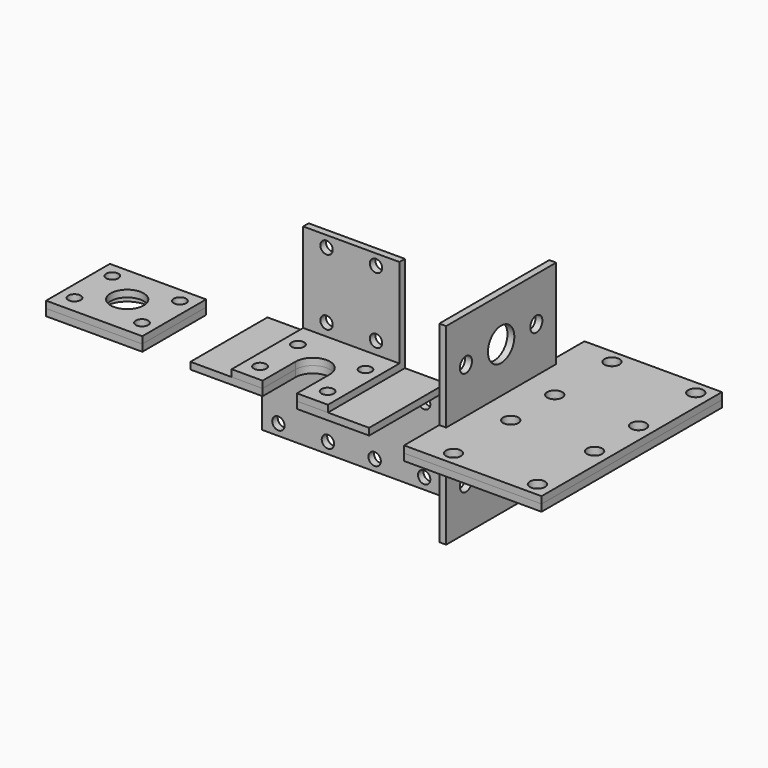
from build123d import *

# Parameters (mm, degrees)
F1_W      = 32.5
F1_H      = 2.5
F1_W_2    = 2.5
F2_DEPTH  = 17.5
F1_H_2    = 32.5
F3_DEPTH  = 17.5
F4_W      = 32.5
F4_H      = 2.5
F4_W_2    = 2.5
F5_DEPTH  = 32.5
F4_H_2    = 32.5
F6_DEPTH  = 32.5
F7_R      = 2.25
F8_DEPTH  = 5
F9_DEPTH  = 5
F11_R     = 2.25
F12_DEPTH = 5
F10_W     = 35
F10_H     = 29
F10_R     = 2.25
F13_DEPTH = 2.5
F14_DEPTH = 2.5
F15_W     = 2.5
F15_H     = 32.5
F15_H_2   = 2.5
F16_DEPTH = 25
F15_W_2   = 47.5
F17_DEPTH = 41
F18_DEPTH = 41
F19_DEPTH = 25
F20_R     = 2.75
F20_R_2   = 6
F21_DEPTH = 2.5
F22_DEPTH = 5
F23_R     = 2.75
F24_DEPTH = 5


with BuildPart() as f2:
    # F1 (on Right) → F2 (new body, symmetric)
    with BuildSketch(Plane.YZ):
        with Locations((-18.75, 1.25)):
            Rectangle(F1_W, F1_H)
        with Locations((-1.25, 1.25)):
            Rectangle(F1_W_2, F1_H)
    extrude(amount=F2_DEPTH, both=True)

    # F1 (on Right) → F3 (join, symmetric)
    with BuildSketch(Plane.YZ):
        with Locations((-1.25, 1.25)):
            Rectangle(F1_W_2, F1_H)
        with Locations((-1.25, 18.75)):
            Rectangle(F1_W_2, F1_H_2)
    extrude(amount=F3_DEPTH, both=True)

    # F7 (on Front) → F8 (cut, symmetric)
    with BuildSketch(Plane.XZ):
        with Locations((9, 31)):
            Circle(F7_R)
        with Locations((9, 7)):
            Circle(F7_R)
        with Locations((-9, 7)):
            Circle(F7_R)
        with Locations((-9, 31)):
            Circle(F7_R)
    extrude(amount=F8_DEPTH, both=True, mode=Mode.SUBTRACT)


with BuildPart() as f5:
    # F4 (on Right) → F5 (new body, symmetric)
    with BuildSketch(Plane.YZ):
        with Locations((-18.75, -1.25)):
            Rectangle(F4_W, F4_H)
        with Locations((-1.25, -1.25)):
            Rectangle(F4_W_2, F4_H)
    extrude(amount=F5_DEPTH, both=True)

    # F4 (on Right) → F6 (join, symmetric)
    with BuildSketch(Plane.YZ):
        with Locations((-1.25, -18.75)):
            Rectangle(F4_W_2, F4_H_2)
        with Locations((-1.25, -1.25)):
            Rectangle(F4_W_2, F4_H)
    extrude(amount=F6_DEPTH, both=True)

    # F7 (on Front) → F9 (cut, symmetric)
    with BuildSketch(Plane.XZ):
        with Locations((26.5, -7)):
            Circle(F7_R)
        with Locations((8.5, -7)):
            Circle(F7_R)
        with Locations((-8.5, -7)):
            Circle(F7_R)
        with Locations((-26.5, -7)):
            Circle(F7_R)
        with Locations((-26.5, -31)):
            Circle(F7_R)
        with Locations((-8.5, -31)):
            Circle(F7_R)
        with Locations((8.5, -31)):
            Circle(F7_R)
        with Locations((26.5, -31)):
            Circle(F7_R)
    extrude(amount=F9_DEPTH, both=True, mode=Mode.SUBTRACT)


with BuildPart() as f12_tool:
    # F11 (on Top) → F12 (new body, symmetric)
    with BuildSketch(Plane.XY):
        with BuildLine():
            ThreePointArc((-6.25, -20), (0, -26.25), (6.25, -20))
            ThreePointArc((6.25, -20), (0, -13.75), (-6.25, -20))
        make_face()
        with BuildLine():
            Line((6.25, -44.9303393665), (6.25, -20))
            ThreePointArc((6.25, -20), (0, -26.25), (-6.25, -20))
            Line((-6.25, -20), (-6.25, -44.9303393665))
            Line((-6.25, -44.9303393665), (6.25, -44.9303393665))
        make_face()
        with Locations((-12.2872806643, -11.3963534547)):
            Circle(F11_R)
        with Locations((12.2872806643, -11.3963534547)):
            Circle(F11_R)
        with Locations((12.2872806643, -28.6036465453)):
            Circle(F11_R)
        with Locations((-12.2872806643, -28.6036465453)):
            Circle(F11_R)
    extrude(amount=F12_DEPTH, both=True)


with BuildPart() as f2_1:
    add(f2.part)

    # F12: cut by f12_tool
    add(f12_tool.part, mode=Mode.SUBTRACT)


with BuildPart() as f5_1:
    add(f5.part)

    # F12: cut by f12_tool
    add(f12_tool.part, mode=Mode.SUBTRACT)


with BuildPart() as f13:
    # F10 (on Top) → F13 (new body)
    with BuildSketch(Plane.XY):
        with Locations((-67.5, -20.5)):
            Rectangle(F10_W, F10_H)
        with BuildLine():
            ThreePointArc((-77.5372806643, -28.6036465453), (-81.9331438035, -29.2802345942), (-77.9441885647, -27.3130995635))
            ThreePointArc((-77.9441885647, -27.3130995635), (-77.6414175252, -27.9270584964), (-77.5372806643, -28.6036465453))
        make_face(mode=Mode.SUBTRACT)
        with Locations((-55.2127193357, -28.6036465453)):
            Circle(F10_R, mode=Mode.SUBTRACT)
        with Locations((-79.7872806643, -11.3963534547)):
            Circle(F10_R, mode=Mode.SUBTRACT)
        with BuildLine():
            ThreePointArc((-74.2580043654, -24.7320055999), (-69.9808228459, -12.1318351563), (-59.25, -20))
            ThreePointArc((-59.25, -20), (-65.0191771541, -27.8681648437), (-74.2580043654, -24.7320055999))
        make_face(mode=Mode.SUBTRACT)
        with Locations((-55.2127193357, -11.3963534547)):
            Circle(F10_R, mode=Mode.SUBTRACT)
    extrude(amount=-F13_DEPTH)


with BuildPart() as f14:
    # F10 (on Top) → F14 (new body)
    with BuildSketch(Plane.XY):
        with Locations((-67.5, -20.5)):
            Rectangle(F10_W, F10_H)
        with BuildLine():
            ThreePointArc((-77.5372806643, -28.6036465453), (-81.9331438035, -29.2802345942), (-77.9441885647, -27.3130995635))
            ThreePointArc((-77.9441885647, -27.3130995635), (-77.6414175252, -27.9270584964), (-77.5372806643, -28.6036465453))
        make_face(mode=Mode.SUBTRACT)
        with Locations((-55.2127193357, -28.6036465453)):
            Circle(F10_R, mode=Mode.SUBTRACT)
        with Locations((-79.7872806643, -11.3963534547)):
            Circle(F10_R, mode=Mode.SUBTRACT)
        with BuildLine():
            ThreePointArc((-74.2580043654, -24.7320055999), (-69.9808228459, -12.1318351563), (-59.25, -20))
            ThreePointArc((-59.25, -20), (-65.0191771541, -27.8681648437), (-74.2580043654, -24.7320055999))
        make_face(mode=Mode.SUBTRACT)
        with Locations((-55.2127193357, -11.3963534547)):
            Circle(F10_R, mode=Mode.SUBTRACT)
        with BuildLine():
            ThreePointArc((-74.2580043654, -24.7320055999), (-65.0191771541, -27.8681648437), (-59.25, -20))
            ThreePointArc((-59.25, -20), (-69.9808228459, -12.1318351563), (-74.2580043654, -24.7320055999))
        make_face()
        with BuildLine():
            ThreePointArc((-61.5, -20), (-65.695765203, -25.7223017045), (-72.4149122657, -23.4414586181))
            ThreePointArc((-72.4149122657, -23.4414586181), (-69.304234797, -14.2776982955), (-61.5, -20))
        make_face(mode=Mode.SUBTRACT)
    extrude(amount=F14_DEPTH)


with BuildPart() as f16:
    # F15 (on Front) → F16 (new body, symmetric)
    with BuildSketch(Plane.XZ):
        with Locations((51.25, -18.75)):
            Rectangle(F15_W, F15_H)
        with Locations((51.25, -1.25)):
            Rectangle(F15_W, F15_H_2)
    extrude(amount=F16_DEPTH, both=True)

    # F15 (on Front) → F17 (join, symmetric)
    with BuildSketch(Plane.XZ):
        with Locations((51.25, -1.25)):
            Rectangle(F15_W, F15_H_2)
        with Locations((76.25, -1.25)):
            Rectangle(F15_W_2, F15_H_2)
    extrude(amount=F17_DEPTH, both=True)

    # F20 (on offset) → F21 (cut, symmetric)
    with BuildSketch(Plane.YZ.offset(50)):
        with Locations((16, -19)):
            Circle(F20_R)
        with Locations((0, -19)):
            Circle(F20_R_2)
        with Locations((-16, -19)):
            Circle(F20_R)
    extrude(amount=F21_DEPTH, both=True, mode=Mode.SUBTRACT)


with BuildPart() as f18:
    # F15 (on Front) → F18 (new body, symmetric)
    with BuildSketch(Plane.XZ):
        with Locations((76.25, 1.25)):
            Rectangle(F15_W_2, F15_H_2)
        with Locations((51.25, 1.25)):
            Rectangle(F15_W, F15_H_2)
    extrude(amount=F18_DEPTH, both=True)

    # F15 (on Front) → F19 (join, symmetric)
    with BuildSketch(Plane.XZ):
        with Locations((51.25, 18.75)):
            Rectangle(F15_W, F15_H)
        with Locations((51.25, 1.25)):
            Rectangle(F15_W, F15_H_2)
    extrude(amount=F19_DEPTH, both=True)

    # F20 (on offset) → F22 (cut, symmetric)
    with BuildSketch(Plane.YZ.offset(50)):
        with Locations((-16, 19)):
            Circle(F20_R)
        with Locations((0, 19)):
            Circle(F20_R_2)
        with Locations((16, 19)):
            Circle(F20_R)
    extrude(amount=F22_DEPTH, both=True, mode=Mode.SUBTRACT)


with BuildPart() as f24_tool:
    # F23 (on Top) → F24 (new body, symmetric)
    with BuildSketch(Plane.XY):
        with Locations((64, -10)):
            Circle(F23_R)
        with Locations((94.5, -10)):
            Circle(F23_R)
        with Locations((94.5, -36)):
            Circle(F23_R)
        with Locations((64, -36)):
            Circle(F23_R)
        with Locations((64, 36)):
            Circle(F23_R)
        with Locations((94.5, 36)):
            Circle(F23_R)
        with Locations((64, 10)):
            Circle(F23_R)
        with Locations((94.5, 10)):
            Circle(F23_R)
    extrude(amount=F24_DEPTH, both=True)


with BuildPart() as f16_1:
    add(f16.part)

    # F24: cut by f24_tool
    add(f24_tool.part, mode=Mode.SUBTRACT)


with BuildPart() as f18_1:
    add(f18.part)

    # F24: cut by f24_tool
    add(f24_tool.part, mode=Mode.SUBTRACT)


solid = Compound([f2_1.part, f5_1.part, f13.part, f14.part, f16_1.part, f18_1.part])
